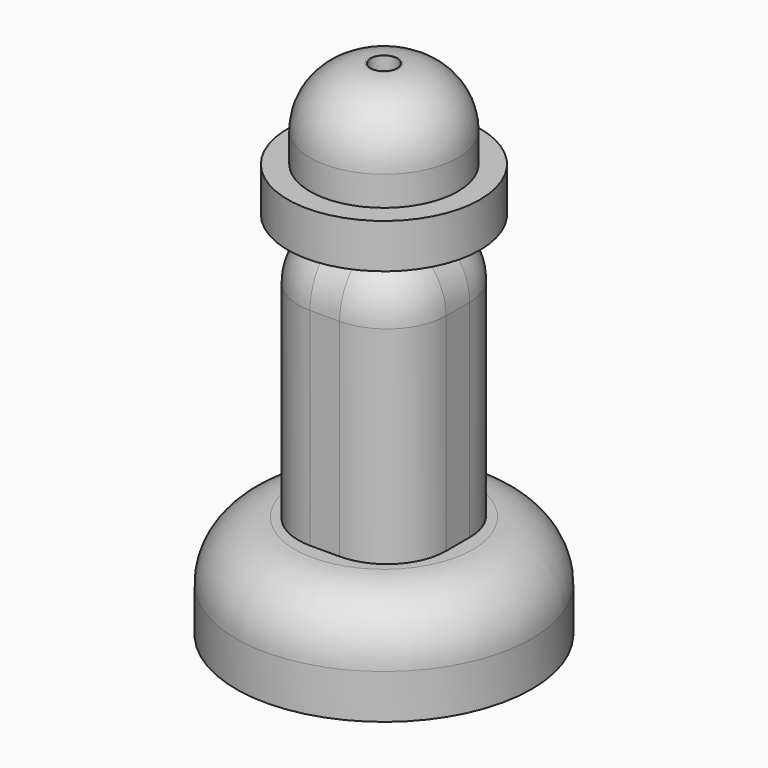
from build123d import *

# Parameters (mm, degrees)
F0_R         = 12.7
F1_DEPTH     = 8.89
F2_W         = 12.7
F2_H         = 12.7
F3_DEPTH     = 31.75
F4_R         = 5.08
F5_T1_DEPTH  = 17.78
F5_S5_W      = 5.08
F5_S5_H      = 5.08
F5_T6_DEPTH  = 5.08
F5_S11_W     = 5.08
F5_S11_H     = 5.08
F5_T12_DEPTH = 5.08
F5_S17_W     = 5.08
F5_S17_H     = 5.08
F5_T18_DEPTH = 5.08
F5_S23_W     = 5.08
F5_S23_H     = 5.08
F5_T24_DEPTH = 5.08
F6_R         = 8.255
F7_DEPTH     = 3.81
F8_R         = 6.35
F9_DEPTH     = 7.62
F10_R        = 5.08
F12_D        = 2.286
F12_DEPTH    = 12.7
F12_TIP      = 0.6867836875
F13_R        = 5.08


# Not quite as in the source:
# - a fillet or chamfer that OpenCascade refuses, or shapes differently, is made with other operations: its cross-section is extruded or revolved along the edge and cut away or added


with BuildPart() as f1:
    # F0 (on Top) → F1 (new body)
    with BuildSketch(Plane.XY):
        Circle(F0_R)
    extrude(amount=F1_DEPTH)

    # F2 (on Top) → F3 (join)
    with BuildSketch(Plane.XY):
        Rectangle(F2_W, F2_H)
    extrude(amount=F3_DEPTH)

    # F4
    f4_edges = [f1.edges().sort_by_distance(p)[0] for p in [
        (6.35, 0, 31.75),
        (0, -6.35, 31.75),
        (-6.35, 0, 31.75),
        (0, 6.35, 31.75),
    ]]
    fillet(f4_edges, radius=F4_R)

    # F5: fillet of radius 5.08 on 4 edges, made by hand

    # F5_s2 → F5_t1 (cut)
    with BuildSketch(Plane.XY.offset(8.89)):
        with BuildLine():
            ThreePointArc((1.27, -6.35), (4.8621024484, -4.8621024484), (6.35, -1.27))
            Line((6.35, -1.27), (6.35, -6.35))
            Line((6.35, -6.35), (1.27, -6.35))
        make_face()
        with BuildLine():
            ThreePointArc((-6.35, -1.27), (-4.8621024484, -4.8621024484), (-1.27, -6.35))
            Line((-1.27, -6.35), (-6.35, -6.35))
            Line((-6.35, -6.35), (-6.35, -1.27))
        make_face()
        with BuildLine():
            ThreePointArc((-6.35, 1.27), (-4.8621024484, 4.8621024484), (-1.27, 6.35))
            Line((-1.27, 6.35), (-6.35, 6.35))
            Line((-6.35, 6.35), (-6.35, 1.27))
        make_face()
        with BuildLine():
            ThreePointArc((1.27, 6.35), (4.8621024484, 4.8621024484), (6.35, 1.27))
            Line((6.35, 1.27), (6.35, 6.35))
            Line((6.35, 6.35), (1.27, 6.35))
        make_face()
    extrude(amount=F5_T1_DEPTH, mode=Mode.SUBTRACT)


with BuildPart() as f5_tool4:
    # F5_s5 → F5_t6 (new body)
    with BuildSketch(Plane.XZ.offset(-1.27)):
        with Locations((3.81, 29.21)):
            Rectangle(F5_S5_W, F5_S5_H)
    extrude(amount=-F5_T6_DEPTH)

    # F5_s7 → F5_t8 (revolve, cut)
    with BuildSketch(Plane(origin=(1.27, 1.27, 26.67), x_dir=(-0.7071067812, 0, -0.7071067812), z_dir=(0.7071067812, 0, -0.7071067812))):
        with BuildLine():
            ThreePointArc((0, -5.08), (5.08, 0), (0, 5.08))
            Line((0, 5.08), (0, -5.08))
        make_face()
    revolve(axis=Axis((1.27, 1.27, 26.67), (0, 1, 0)), mode=Mode.SUBTRACT)


with BuildPart() as f1_1:
    add(f1.part)

    # F5_t3: cut F5_tool4
    add(f5_tool4.part, mode=Mode.SUBTRACT)


with BuildPart() as f5_tool10:
    # F5_s11 → F5_t12 (new body)
    with BuildSketch(Plane.YZ.offset(-1.27)):
        with Locations((3.81, 29.21)):
            Rectangle(F5_S11_W, F5_S11_H)
    extrude(amount=-F5_T12_DEPTH)

    # F5_s13 → F5_t14 (revolve, cut)
    with BuildSketch(Plane(origin=(-1.27, 1.27, 26.67), x_dir=(0, -0.7071067812, -0.7071067812), z_dir=(0, 0.7071067812, -0.7071067812))):
        with BuildLine():
            ThreePointArc((0, -5.08), (5.08, 0), (0, 5.08))
            Line((0, 5.08), (0, -5.08))
        make_face()
    revolve(axis=Axis((-1.27, 1.27, 26.67), (-1, 0, 0)), mode=Mode.SUBTRACT)


with BuildPart() as f1_2:
    add(f1_1.part)

    # F5_t9: cut F5_tool10
    add(f5_tool10.part, mode=Mode.SUBTRACT)


with BuildPart() as f5_tool16:
    # F5_s17 → F5_t18 (new body)
    with BuildSketch(Plane.YZ.offset(-1.27)):
        with Locations((-3.81, 29.21)):
            Rectangle(F5_S17_W, F5_S17_H)
    extrude(amount=-F5_T18_DEPTH)

    # F5_s19 → F5_t20 (revolve, cut)
    with BuildSketch(Plane(origin=(-1.27, -1.27, 26.67), x_dir=(0, 0.7071067812, -0.7071067812), z_dir=(0, 0.7071067812, 0.7071067812))):
        with BuildLine():
            ThreePointArc((0, -5.08), (5.08, 0), (0, 5.08))
            Line((0, 5.08), (0, -5.08))
        make_face()
    revolve(axis=Axis((-1.27, -1.27, 26.67), (-1, 0, 0)), mode=Mode.SUBTRACT)


with BuildPart() as f1_3:
    add(f1_2.part)

    # F5_t15: cut F5_tool16
    add(f5_tool16.part, mode=Mode.SUBTRACT)


with BuildPart() as f5_tool22:
    # F5_s23 → F5_t24 (new body)
    with BuildSketch(Plane.XZ.offset(1.27)):
        with Locations((3.81, 29.21)):
            Rectangle(F5_S23_W, F5_S23_H)
    extrude(amount=F5_T24_DEPTH)

    # F5_s25 → F5_t26 (revolve, cut)
    with BuildSketch(Plane(origin=(1.27, -1.27, 26.67), x_dir=(-0.7071067812, 0, -0.7071067812), z_dir=(-0.7071067812, 0, 0.7071067812))):
        with BuildLine():
            ThreePointArc((0, -5.08), (5.08, 0), (0, 5.08))
            Line((0, 5.08), (0, -5.08))
        make_face()
    revolve(axis=Axis((1.27, -1.27, 26.67), (0, -1, 0)), mode=Mode.SUBTRACT)


with BuildPart() as f1_4:
    add(f1_3.part)

    # F5_t21: cut F5_tool22
    add(f5_tool22.part, mode=Mode.SUBTRACT)

    # F6 (on face) → F7 (join)
    with BuildSketch(Plane.XY.offset(31.75)):
        Circle(F6_R)
    extrude(amount=F7_DEPTH)

    # F8 (on face) → F9 (join)
    with BuildSketch(Plane.XY.offset(35.56)):
        Circle(F8_R)
    extrude(amount=F9_DEPTH)

    # F10
    f10_edges = [f1_4.edges().sort_by_distance(p)[0] for p in [
        (-6.35, 0, 43.18),
    ]]
    fillet(f10_edges, radius=F10_R)

    # F12
    with Locations(Plane.XY.offset(43.18)):
        with Locations((0, 0)):
            Hole(F12_D / 2, depth=F12_DEPTH)
            with Locations((0, 0, -(F12_DEPTH + F12_TIP / 2))):  # 118° drill point
                Cone(0, F12_D / 2, F12_TIP, mode=Mode.SUBTRACT)

    # F13
    f13_edges = [f1_4.edges().sort_by_distance(p)[0] for p in [
        (-12.7, 0, 8.89),
    ]]
    fillet(f13_edges, radius=F13_R)


solid = f1_4.part
